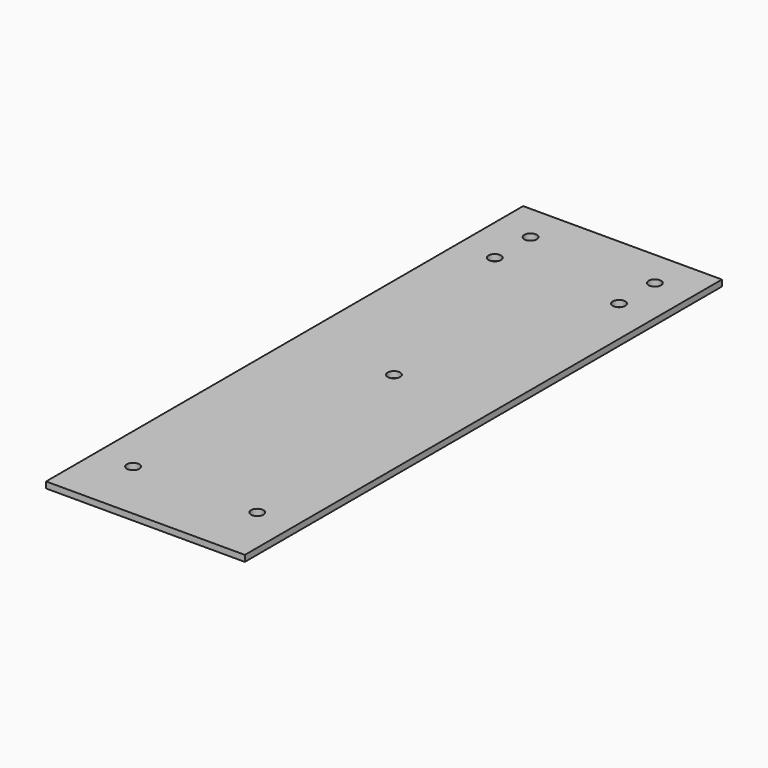
from build123d import *

# Parameters (mm, degrees)
F0_W     = 101.6
F0_H     = 304.8
F1_DEPTH = 3.175
F3_D     = 6.35


# Not quite as in the source:
# - a length typed as a fraction of an inch, garbled in the dataset ("3 / 203.2 mm" for 3/8 in), is restored


with BuildPart() as f1:
    # F0 (on Top) → F1 (new body)
    with BuildSketch(Plane.XY):
        Rectangle(F0_W, F0_H)
    extrude(amount=F1_DEPTH)

    # F3 (through all)
    with Locations(Plane.XY.offset(3.175)):
        with Locations((-31.75, 133.35), (31.75, 133.35), (31.75, -120.65), (-31.75, -120.65), (0, 6.35), (-31.75, 110.49), (31.75, 110.49)):
            Hole(F3_D / 2)


solid = f1.part
